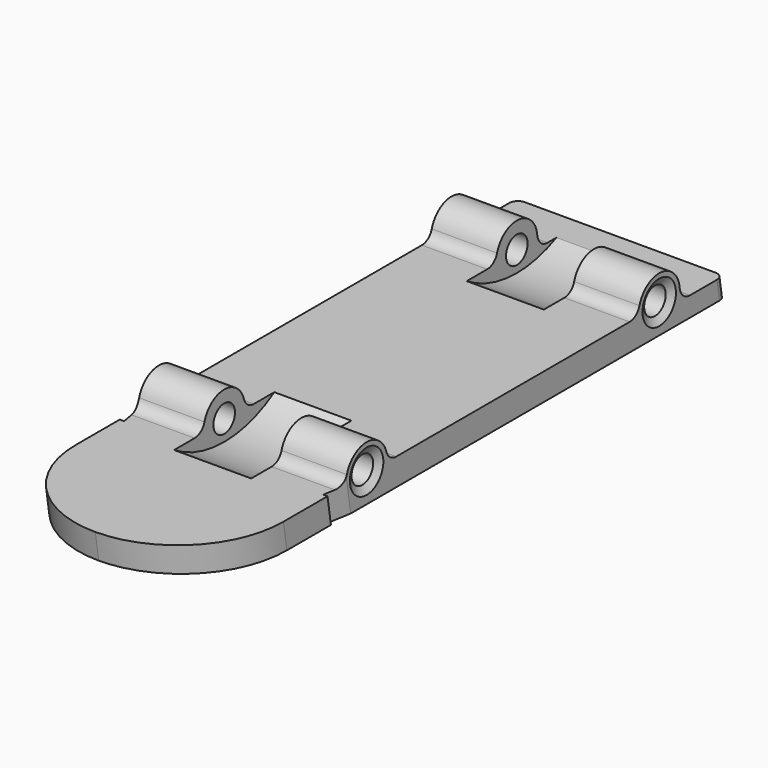
from build123d import *

# Parameters (mm, degrees)
F0_R        = 0.8001
F1_DEPTH    = 6.1595
F2_R        = 0.762
F3_SIZE2    = 0.4399409051
F3_SIZE     = 0.254
F3_2_SIZE2  = 0.4399409051
F3_2_SIZE   = 0.254
F4_SIZE2    = 0.4399409051
F4_SIZE     = 0.254
F6_DEPTH    = 2.286
F8_R        = 0.508
F9_T1_DEPTH = 32.4811466943
F11_DEPTH   = 12.7


# Not quite as in the source:
# - a fillet or chamfer that OpenCascade refuses, or shapes differently, is made with other operations: its cross-section is extruded or revolved along the edge and cut away or added


with BuildPart() as f1:
    # F0 (on Right) → F1 (new body, symmetric)
    with BuildSketch(Plane.YZ):
        with BuildLine():
            Line((-19.6694904986, 1.6002), (-19.4160437172, 0))
            Line((-19.4160437172, 0), (19.4160437172, 0))
            Line((19.4160437172, 0), (19.2309873372, 1.1684))
            Line((19.2309873372, 1.1684), (15.8541987451, 1.1684))
            ThreePointArc((15.8541987451, 1.1684), (14.6580511896, 3.2349867583), (12.9176425998, 1.6002))
            Line((12.9176425998, 1.6002), (-5.7365591714, 1.6002))
            ThreePointArc((-5.7365591714, 1.6002), (-7.2552582858, 3.2512), (-8.7739574002, 1.6002))
            Line((-8.7739574002, 1.6002), (-19.6694904986, 1.6002))
        make_face()
        with Locations((-7.2552582858, 1.7272)):
            Circle(F0_R, mode=Mode.SUBTRACT)
        with Locations((14.4363417142, 1.7272)):
            Circle(F0_R, mode=Mode.SUBTRACT)
    extrude(amount=F1_DEPTH, both=True)

    # F2
    f2_edges = [f1.edges().sort_by_distance(p)[0] for p in [
        (0, -8.773957, 1.6002),
        (0, -5.736559, 1.6002),
        (0, 12.917643, 1.6002),
        (0, 15.854199, 1.1684),
    ]]
    fillet(f2_edges, radius=F2_R)

    # F3
    f3_edges = [f1.edges().sort_by_distance(p)[0] for p in [
        (6.1595, -8.055358, 1.7272),
        (-6.1595, -8.055358, 1.7272),
    ]]
    f3_side = f1.faces().sort_by_distance((0, -8.055358, 1.7272))[0]
    chamfer(f3_edges, length=F3_SIZE, length2=F3_SIZE2, reference=f3_side)

    # F3#2
    f3_2_edges = [f1.edges().sort_by_distance(p)[0] for p in [
        (6.1595, 13.636242, 1.7272),
    ]]
    f3_2_side = f1.faces().sort_by_distance((0, 13.636242, 1.7272))[0]
    chamfer(f3_2_edges, length=F3_2_SIZE, length2=F3_2_SIZE2, reference=f3_2_side)

    # F4
    f4_edges = [f1.edges().sort_by_distance(p)[0] for p in [
        (-6.1595, 13.636242, 1.7272),
    ]]
    f4_side = f1.faces().sort_by_distance((-0.127, 13.636242, 1.7272))[0]
    chamfer(f4_edges, length=F4_SIZE, length2=F4_SIZE2, reference=f4_side)

    # F5 (on Right) → F6 (cut, symmetric)
    with BuildSketch(Plane.YZ):
        with BuildLine():
            Line((-1.4272936791, 3.7511704683), (-13.4970735674, 4.5248900073))
            ThreePointArc((-13.4970735674, 4.5248900073), (-7.6939820902, 0.5220475291), (-1.4272936791, 3.7511704683))
        make_face()
        with BuildLine():
            Line((20.2263604549, 3.6906977019), (8.6020119823, 3.7614527913))
            ThreePointArc((8.6020119823, 3.7614527913), (14.3945992101, 0.508127038), (20.2263604549, 3.6906977019))
        make_face()
    extrude(amount=F6_DEPTH, both=True, mode=Mode.SUBTRACT)

    # F8
    f8_edges = [f1.edges().sort_by_distance(p)[0] for p in [
        (6.1595, 19.323516, 0.5842),
        (-6.1595, 19.323516, 0.5842),
    ]]
    fillet(f8_edges, radius=F8_R)

    # F9: fillet of radius 6.1722 on 2 edges, made by hand

    # F9_s2 → F9_t1 (cut)
    with BuildSketch(Plane(origin=(0, -3.1424532039, 19.8406686756), x_dir=(1, 0, 0), z_dir=(0, 0.156434465, -0.9876883406))):
        with BuildLine():
            ThreePointArc((6.1595, 13.0048), (4.3517044748, 17.3692044748), (-0.0127, 19.177))
            Line((-0.0127, 19.177), (6.1595, 19.177))
            Line((6.1595, 19.177), (6.1595, 13.0048))
        make_face()
        with BuildLine():
            ThreePointArc((0.0127, 19.177), (-4.3517044748, 17.3692044748), (-6.1595, 13.0048))
            Line((-6.1595, 13.0048), (-6.1595, 19.177))
            Line((-6.1595, 19.177), (0.0127, 19.177))
        make_face()
    extrude(amount=F9_T1_DEPTH, mode=Mode.SUBTRACT)

    # F10 (on line) → F11 (cut, symmetric)
    with BuildSketch(Plane(origin=(0, -0.4444158842, 2.8059314619), x_dir=(1, 0, 0), z_dir=(0, -0.156434465, 0.9876883406))):
        Polygon((5.9055, -9.7789869341), (6.1595, -9.7789869341), (6.1595, -8.338481352), align=None)
        Polygon((-6.1595, -8.338481352), (-6.1595, -9.7789869341), (-5.9055, -9.7789869341), align=None)
    extrude(amount=F11_DEPTH, both=True, mode=Mode.SUBTRACT)


solid = f1.part
